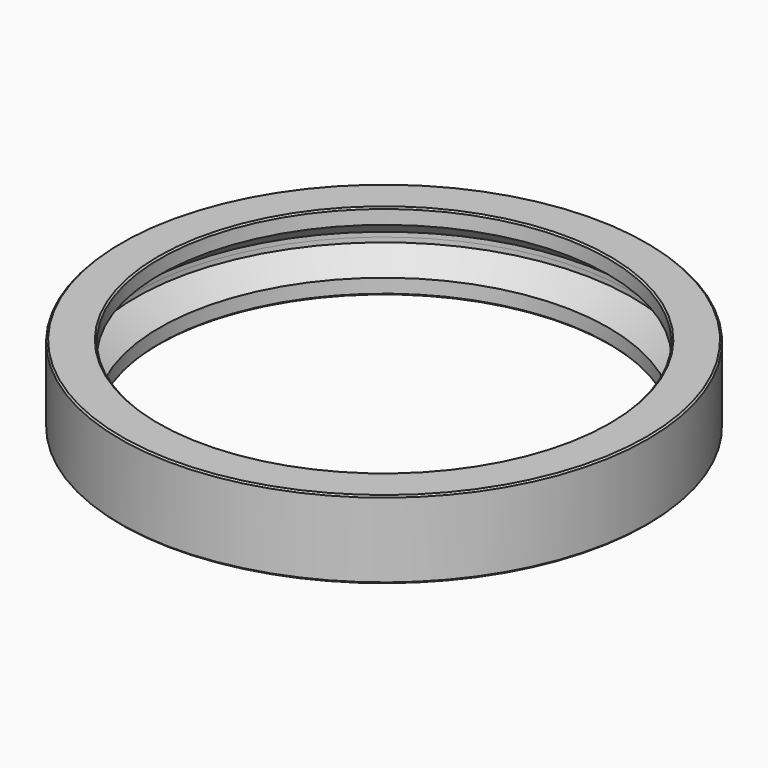
from build123d import *

# Parameters (mm, degrees)
F0_R          = 17
F0_R_2        = 16
F0_R_3        = 14.45
F1_DEPTH      = 2.5
F2_DEPTH      = 1.5
F2_DEPTH_BACK = 1.5
F3_SIZE2      = 1.19999
F3_SIZE       = 1.54999
F4_SIZE       = 0.1
F6_SIZE       = 0.1


# Not quite as in the source:
# - a fillet or chamfer is up to 0.001 mm smaller than in the source, because OpenCascade refuses the exact size


with BuildPart() as f1:
    # F0 (on Top) → F1 (new body, symmetric)
    with BuildSketch(Plane.XY):
        Circle(F0_R)
        Circle(F0_R_2, mode=Mode.SUBTRACT)
        Circle(F0_R_2)
        Circle(F0_R_3, mode=Mode.SUBTRACT)
    extrude(amount=F1_DEPTH, both=True)

    # F0 (on Top) → F2 (cut, two sides)
    with BuildSketch(Plane.XY) as f2_sk:
        Circle(F0_R_2)
        Circle(F0_R_3, mode=Mode.SUBTRACT)
    extrude(amount=F2_DEPTH, mode=Mode.SUBTRACT)
    extrude(f2_sk.sketch, amount=-F2_DEPTH_BACK, mode=Mode.SUBTRACT)

    # F3 (size 1.55 and 1.2 in the source; OpenCascade refuses exactly that, so slightly less here)
    f3_edges = [f1.edges().sort_by_distance(p)[0] for p in [
        (-16, 0, -1.5),
        (-16, 0, 1.5),
    ]]
    chamfer(f3_edges, length=F3_SIZE, length2=F3_SIZE2)

    # F4
    f4_edges = [f1.edges().sort_by_distance(p)[0] for p in [
        (-17, 0, 2.5),
        (-17, 0, -2.5),
    ]]
    chamfer(f4_edges, length=F4_SIZE)

    # F6
    f6_edges = [f1.edges().sort_by_distance(p)[0] for p in [
        (-14.45, 0, 2.5),
        (-14.45, 0, -2.5),
    ]]
    chamfer(f6_edges, length=F6_SIZE)


solid = f1.part
